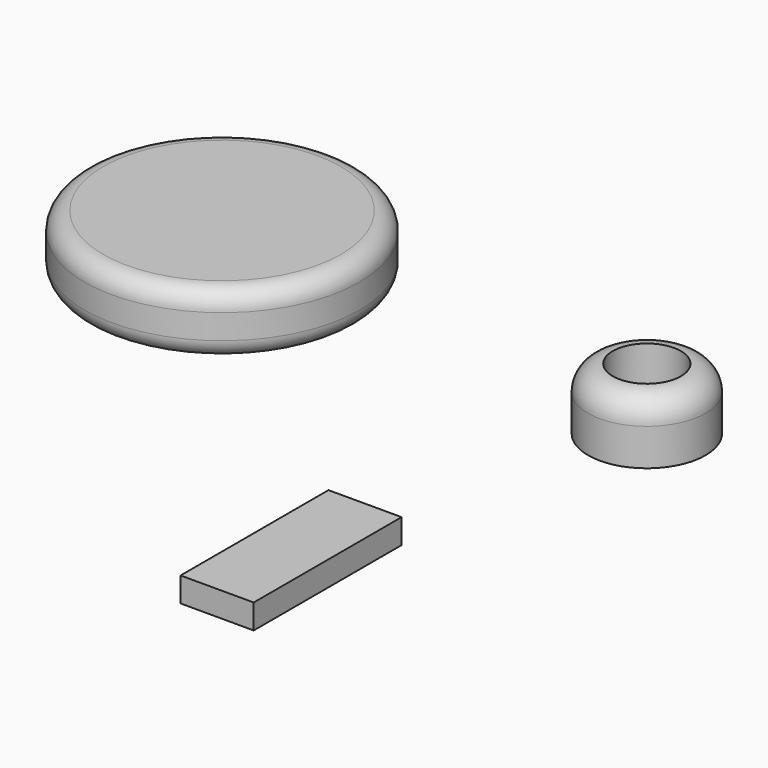
from build123d import *

# Parameters (mm, degrees)
F0_W     = 59.3491444241
F0_H     = 150
F1_DEPTH = 20
F2_R     = 47.6583720873
F3_DEPTH = 50
F4_R     = 20
F5_T     = -20
F6_R     = 111.5009996007
F7_DEPTH = 50
F8_R     = 15
F9_R     = 15


# Not quite as in the source:
# - a shell that OpenCascade refuses in one call is made with other operations: the cavity is built on its own and cut out


with BuildPart() as f1:
    # F0 (on Top) → F1 (new body)
    with BuildSketch(Plane.XY):
        with Locations((-143.2152688503, -324.6246539056)):
            Rectangle(F0_W, F0_H)
    extrude(amount=-F1_DEPTH)


with BuildPart() as f3:
    # F2 (on Top) → F3 (new body)
    with BuildSketch(Plane.XY):
        with Locations((-63.7783035636, -63.0468800664)):
            Circle(F2_R)
    extrude(amount=F3_DEPTH)

    # F4
    f4_edges = [f3.edges().sort_by_distance(p)[0] for p in [
        (-111.436676, -63.04688, 50),
    ]]
    fillet(f4_edges, radius=F4_R)

    # F5: a shell. OpenCascade refuses it in one call, so the cavity is built on its own and cut out:
    # the body offset inwards by the wall thickness, plus a prism from it out through each open face.
    f5_core = offset(f3.part, amount=F5_T, kind=Kind.INTERSECTION, mode=Mode.PRIVATE)
    f5_exits = [f5_core.faces().sort_by_distance(p)[0] for p in [
        (-63.778304, -63.04688, 30),
    ]]
    add(f5_core, mode=Mode.SUBTRACT)
    extrude(f5_exits, amount=-F5_T, mode=Mode.SUBTRACT)


with BuildPart() as f7:
    # F6 (on Top) → F7 (new body)
    with BuildSketch(Plane.XY):
        with Locations((-405.2630662918, -67.0995116234)):
            Circle(F6_R)
    extrude(amount=F7_DEPTH)

    # F8
    f8_edges = [f7.edges().sort_by_distance(p)[0] for p in [
        (-516.764066, -67.099512, 50),
    ]]
    fillet(f8_edges, radius=F8_R)

    # F9
    f9_edges = [f7.edges().sort_by_distance(p)[0] for p in [
        (-516.764066, -67.099512, 0),
    ]]
    fillet(f9_edges, radius=F9_R)


solid = Compound([f1.part, f3.part, f7.part])
